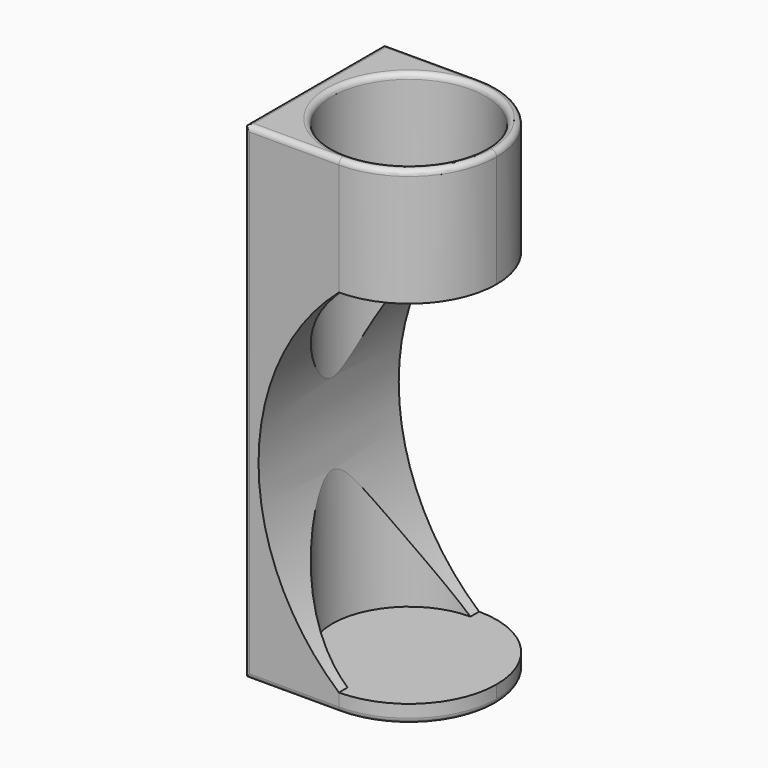
from build123d import *

# Parameters (mm, degrees)
F1_DEPTH      = 135
F2_R          = 21.25
F3_DEPTH      = 130
F4_W          = 24.25
F4_H          = 97.5
F5_DEPTH      = 50.1
F5_DEPTH_BACK = 25
F6_R          = 1.49999
F7_T3_DEPTH   = 141.00001
F7_T6_DEPTH   = 56
F7_T9_DEPTH   = 141.00001
F8_T1_DEPTH   = 28.5
F8_T4_ANGLE   = 180


# Not quite as in the source:
# - a fillet or chamfer that OpenCascade refuses, or shapes differently, is made with other operations: its cross-section is extruded or revolved along the edge and cut away or added
# - a fillet or chamfer is up to 0.001 mm smaller than in the source, because OpenCascade refuses the exact size


with BuildPart() as f1:
    # F0 (on Top) → F1 (new body)
    with BuildSketch(Plane.XY):
        with BuildLine():
            ThreePointArc((0, -24.25), (17.1473394438, -17.1473394438), (24.25, 0))
            ThreePointArc((24.25, 0), (17.1473394438, 17.1473394438), (0, 24.25))
            ThreePointArc((0, 24.25), (-24.25, 0), (0, -24.25))
        make_face()
        with BuildLine():
            ThreePointArc((0, -24.25), (-24.25, 0), (0, 24.25))
            Line((0, 24.25), (-26.25, 24.25))
            Line((-26.25, 24.25), (-26.25, -24.25))
            Line((-26.25, -24.25), (0, -24.25))
        make_face()
    extrude(amount=-F1_DEPTH)

    # F2 (on face) → F3 (cut)
    with BuildSketch(Plane.XY):
        Circle(F2_R)
    extrude(amount=-F3_DEPTH, mode=Mode.SUBTRACT)

    # F4 (on face) → F5 (cut, two sides)
    with BuildSketch(Plane.XZ.offset(24.25)) as f5_sk:
        with Locations((12.125, -81.25)):
            Rectangle(F4_W, F4_H)
        with BuildLine():
            Line((0, -130), (0, -32.5))
            ThreePointArc((0, -32.5), (-22.2460263089, -81.25), (0, -130))
        make_face()
    extrude(amount=-F5_DEPTH, mode=Mode.SUBTRACT)
    extrude(f5_sk.sketch, amount=F5_DEPTH_BACK, mode=Mode.SUBTRACT)

    # F6 (radius 1.5 in the source; OpenCascade refuses exactly that, so slightly less here)
    f6_edges = [f1.edges().sort_by_distance(p)[0] for p in [
        (24.25, 0, 0),
        (-13.125, -24.25, 0),
        (-13.125, 24.25, 0),
        (-26.25, 0, 0),
        (-21.25, 0, 0),
    ]]
    fillet(f6_edges, radius=F6_R)

    # F7: fillet of radius 1.5 on 4 edges, made by hand


with BuildPart() as f7_tool1:
    # F7_s2 → F7_t3 (new body)
    with BuildSketch(Plane.XY.offset(2.25001)):
        with BuildLine():
            ThreePointArc((-24.75, 24.25), (-25.8106601718, 23.8106601718), (-26.25, 22.75))
            Line((-26.25, 22.75), (-26.25, 24.25))
            Line((-26.25, 24.25), (-24.75, 24.25))
        make_face()
    extrude(amount=-F7_T3_DEPTH)


with BuildPart() as f7_tool4:
    # F7_s5 → F7_t6 (new body)
    with BuildSketch(Plane.XZ.offset(-28)):
        with BuildLine():
            ThreePointArc((-26.25, -133.5), (-25.8106601718, -134.5606601718), (-24.75, -135))
            Line((-24.75, -135), (-26.25, -135))
            Line((-26.25, -135), (-26.25, -133.5))
        make_face()
    extrude(amount=F7_T6_DEPTH)


with BuildPart() as f7_tool7:
    # F7_s8 → F7_t9 (new body)
    with BuildSketch(Plane.XY.offset(2.25001)):
        with BuildLine():
            ThreePointArc((-24.75, -24.25), (-25.8106601718, -23.8106601718), (-26.25, -22.75))
            Line((-26.25, -22.75), (-26.25, -24.25))
            Line((-26.25, -24.25), (-24.75, -24.25))
        make_face()
    extrude(amount=-F7_T9_DEPTH)


with BuildPart() as f1_1:
    add(f1.part)

    # F7_t10: cut F7_tool1, F7_tool4, F7_tool7
    add([f7_tool1.part, f7_tool4.part, f7_tool7.part], mode=Mode.SUBTRACT)

    # F8: fillet of radius 1.5 on 4 edges, made by hand

    # F8_s2 → F8_t1 (cut)
    with BuildSketch(Plane.YZ.offset(-28.5)):
        with BuildLine():
            ThreePointArc((-24.25, -133.5), (-23.8106601718, -134.5606601718), (-22.75, -135))
            Line((-22.75, -135), (-24.25, -135))
            Line((-24.25, -135), (-24.25, -133.5))
        make_face()
        with BuildLine():
            ThreePointArc((24.25, -133.5), (23.8106601718, -134.5606601718), (22.75, -135))
            Line((22.75, -135), (24.25, -135))
            Line((24.25, -135), (24.25, -133.5))
        make_face()
    extrude(amount=F8_T1_DEPTH, mode=Mode.SUBTRACT)

    # F8_s3 → F8_t4 (revolve, cut)
    with BuildSketch(Plane.YZ):
        with BuildLine():
            ThreePointArc((-24.25, -133.5), (-23.8106601718, -134.5606601718), (-22.75, -135))
            Line((-22.75, -135), (-24.25, -135))
            Line((-24.25, -135), (-24.25, -133.5))
        make_face()
    revolve(axis=Axis((0, 0, -135), (0, 0, 1)), revolution_arc=F8_T4_ANGLE, mode=Mode.SUBTRACT)


solid = f1_1.part
